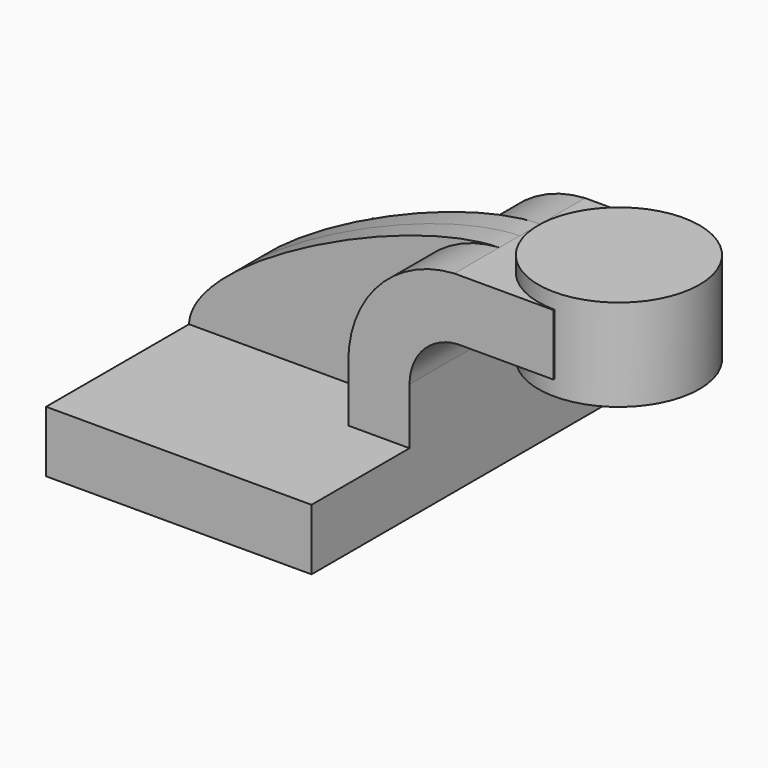
from build123d import *

# Parameters (mm, degrees)
F1_DEPTH = 63.5
F0_W     = 25.7461559653
F0_H     = 19.0207560397
F2_DEPTH = 25.4
F3_DEPTH = 7.9375


# Not quite as in the source:
# - a feature names something its author has since deleted; it is built from what else it names


with BuildPart() as f1:
    # F0 (on Front) → F1 (new body, symmetric)
    with BuildSketch(Plane.XZ):
        Polygon((22.225, 9.525), (-41.275, 9.525), (-41.275, -9.525), (41.275, -9.525), (41.275, 9.525), align=None)
    extrude(amount=F1_DEPTH, both=True)

    # F0 (on Front) → F2 (join, symmetric)
    with BuildSketch(Plane.XZ):
        with BuildLine():
            Line((22.225, 27.0245699669), (22.225, 9.525))
            Line((22.225, 9.525), (41.275, 9.525))
            Line((41.275, 9.525), (41.275, 27.0245699669))
            ThreePointArc((41.275, 27.0245699669), (45.6179930488, 37.9345855799), (56.2707090616, 42.8752))
            Line((56.2707090616, 42.8752), (60.325, 42.8752))
            Line((60.325, 42.8752), (60.325, 61.8959560397))
            Line((60.325, 61.8959560397), (55.2155599356, 61.8959560397))
            ThreePointArc((55.2155599356, 61.8959560397), (31.7795847073, 51.0266043156), (22.225, 27.0245699669))
        make_face()
        with Locations((73.1980779827, 52.3855780199)):
            Rectangle(F0_W, F0_H)
    extrude(amount=F2_DEPTH, both=True)

    # F0 (on Front) → F3 (join, symmetric)
    with BuildSketch(Plane.XZ):
        with BuildLine():
            add(Edge.make_bspline(
                [(-41.275, 9.525), (-40.530513972, 29.3039940298), (25.5654975772, 61.4196136594), (55.2155599356, 61.8959560397)],
                knots=[0, 0, 0, 0, 109.7868170282, 109.7868170282, 109.7868170282, 109.7868170282], degree=3))
            Line((-41.275, 9.525), (22.225, 9.525))
            Line((22.225, 9.525), (22.225, 27.0245699669))
            ThreePointArc((22.225, 27.0245699669), (31.7795847073, 51.0266043156), (55.2155599356, 61.8959560397))
        make_face()
    extrude(amount=F3_DEPTH, both=True)

    # F0 (on Front) → F4 (revolve)
    with BuildSketch(Plane.XZ):
        Polygon((86.0711559653, 66.675), (86.0711559653, 61.8959560397), (86.0711559653, 42.8752), (86.0711559653, 38.1), (111.125, 38.1), (111.125, 66.675), align=None)
    revolve(axis=Axis((86.0711559653, 0, 52.3875), (0, 0, 1)))


solid = f1.part
